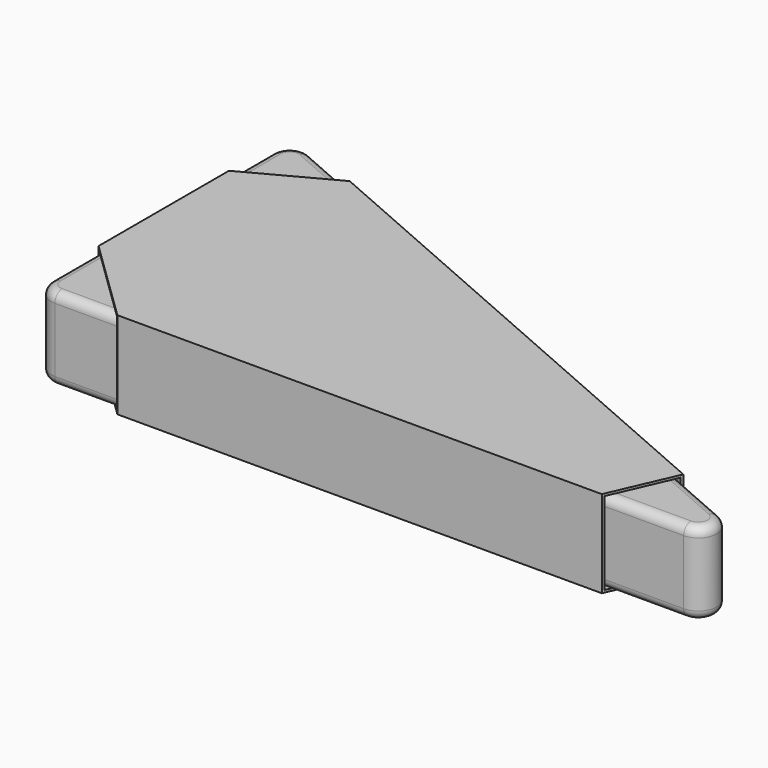
from build123d import *

# Parameters (mm, degrees)
F2_DEPTH = 18
F3_START = 18
F3_DEPTH = 0.5
F4_DEPTH = 0.5
F5_DEPTH = 18
F6_R     = 4
F7_R     = 2


with BuildPart() as f2:
    # F0 (on Top) → F2 (new body)
    with BuildSketch(Plane.XY):
        Polygon((63.5371690989, -29.7485813498), (-96.4628309011, 40.2514186502), (-96.4628309011, -29.7485813498), align=None)
    extrude(amount=F2_DEPTH)

    # F6
    f6_edges = [f2.edges().sort_by_distance(p)[0] for p in [
        (63.537169, -29.748581, 9),
        (-96.462831, 40.251419, 9),
        (-96.462831, -29.748581, 9),
    ]]
    fillet(f6_edges, radius=F6_R)

    # F7
    f7_edges = [f2.edges().sort_by_distance(p)[0] for p in [
        (-96.462831, 4.193388, 18),
        (-24.024045, -29.748581, 18),
        (-95.291258, -28.577008, 18),
        (48.330001, -26.567569, 18),
        (-22.42077, 7.858017, 18),
        (-94.652226, 37.482975, 18),
        (-22.42077, 7.858017, 0),
        (-94.652226, 37.482975, 0),
        (-96.462831, 4.193388, 0),
        (-95.291258, -28.577008, 0),
        (-24.024045, -29.748581, 0),
        (48.330001, -26.567569, 0),
    ]]
    fillet(f7_edges, radius=F7_R)


with BuildPart() as f3:
    # F1 (on Top) → F3 (new body)
    with BuildSketch(Plane.XY.offset(F3_START)):
        Polygon((27.2303114762, -29.7686234117), (-78.958476275, -29.7686234117), (-78.4439082405, -30.2686234117), (27.0115614762, -30.2686234117), align=None)
        Polygon((-78.4439082405, 32.9444158173), (-79.0047962132, 32.644046518), (33.0817828051, -16.3938318026), (33.2821922221, -15.9357531351), align=None)
        Polygon((-79.0047962132, 32.644046518), (-96.3472649455, 23.3567281295), (-96.3472649455, -12.8721320786), (-78.958476275, -29.7686234117), (27.2303114762, -29.7686234117), (33.0817828051, -16.3938318026), align=None)
        Polygon((-96.3472649455, -12.8721320786), (-96.3472649455, 23.3567281295), (-96.8472649455, 23.0889658365), (-96.8472649455, -12.3862876747), align=None)
    extrude(amount=F3_DEPTH)



with BuildPart() as f4:
    # F1 (on Top) → F4 (new body)
    with BuildSketch(Plane.XY):
        Polygon((-79.0047962132, 32.644046518), (-96.3472649455, 23.3567281295), (-96.3472649455, -12.8721320786), (-78.958476275, -29.7686234117), (27.2303114762, -29.7686234117), (33.0817828051, -16.3938318026), align=None)
        Polygon((-96.3472649455, -12.8721320786), (-96.3472649455, 23.3567281295), (-96.8472649455, 23.0889658365), (-96.8472649455, -12.3862876747), align=None)
        Polygon((-78.4439082405, 32.9444158173), (-79.0047962132, 32.644046518), (33.0817828051, -16.3938318026), (33.2821922221, -15.9357531351), align=None)
        Polygon((27.2303114762, -29.7686234117), (-78.958476275, -29.7686234117), (-78.4439082405, -30.2686234117), (27.0115614762, -30.2686234117), align=None)
    extrude(amount=-F4_DEPTH)


with BuildPart() as f3_1:
    add(f3.part)

    add(f4.part)  # F5 merges F4
    # F1 (on Top) → F5 (join)
    with BuildSketch(Plane.XY):
        Polygon((-78.4439082405, 32.9444158173), (-79.0047962132, 32.644046518), (33.0817828051, -16.3938318026), (33.2821922221, -15.9357531351), align=None)
        Polygon((-96.3472649455, -12.8721320786), (-96.3472649455, 23.3567281295), (-96.8472649455, 23.0889658365), (-96.8472649455, -12.3862876747), align=None)
        Polygon((27.2303114762, -29.7686234117), (-78.958476275, -29.7686234117), (-78.4439082405, -30.2686234117), (27.0115614762, -30.2686234117), align=None)
    extrude(amount=F5_DEPTH)


solid = Compound([f2.part, f3_1.part])
